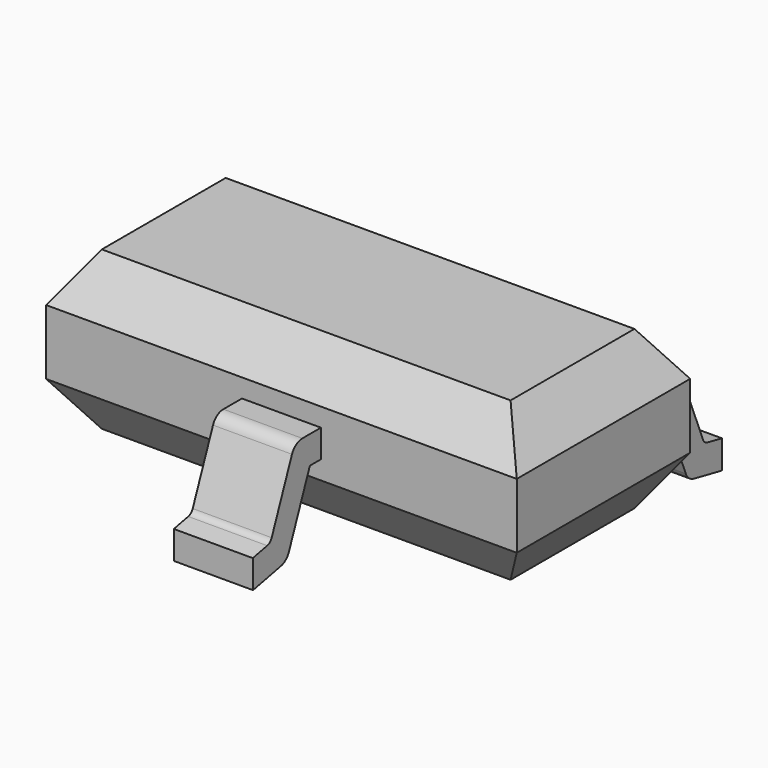
from build123d import *

# Parameters (mm, degrees)
F1_W       = 3.04
F1_H       = 1.4
F2_DEPTH   = 1.02
F3_SIZE2   = 0.3
F3_SIZE    = 0.2
F3_2_SIZE2 = 0.3
F3_2_SIZE  = 0.2
F4_SIZE2   = 0.3
F4_SIZE    = 0.2
F4_2_SIZE2 = 0.3
F4_2_SIZE  = 0.2
F10_DEPTH  = 0.255
F13_DEPTH  = 0.255


# Not quite as in the source:
# - a pattern or mirror of a feature is missing from the dataset's text; its kind, count and spacing are read off the source's solid


with BuildPart() as f2:
    # F1 (on offset) → F2 (new body)
    with BuildSketch(Plane.XY.offset(0.1)):
        Rectangle(F1_W, F1_H)
    extrude(amount=F2_DEPTH)

    # F3
    f3_edges = [f2.edges().sort_by_distance(p)[0] for p in [
        (-1.52, 0, 1.12),
        (1.52, 0, 1.12),
    ]]
    f3_side = f2.faces().sort_by_distance((0, 0, 1.12))[0]
    chamfer(f3_edges, length=F3_SIZE, length2=F3_SIZE2, reference=f3_side)

    # F3#2
    f3_2_edges = [f2.edges().sort_by_distance(p)[0] for p in [
        (-1.52, 0, 0.1),
        (1.52, 0, 0.1),
    ]]
    f3_2_side = f2.faces().sort_by_distance((0, 0, 0.1))[0]
    chamfer(f3_2_edges, length=F3_2_SIZE, length2=F3_2_SIZE2, reference=f3_2_side)

    # F4
    f4_edges = [f2.edges().sort_by_distance(p)[0] for p in [
        (0, -0.7, 1.12),
        (0, 0.7, 1.12),
    ]]
    f4_side = f2.faces().sort_by_distance((0, 0, 1.12))[0]
    chamfer(f4_edges, length=F4_SIZE, length2=F4_SIZE2, reference=f4_side)

    # F4#2
    f4_2_edges = [f2.edges().sort_by_distance(p)[0] for p in [
        (0, -0.7, 0.1),
        (0, 0.7, 0.1),
    ]]
    f4_2_side = f2.faces().sort_by_distance((0, 0, 0.1))[0]
    chamfer(f4_2_edges, length=F4_2_SIZE, length2=F4_2_SIZE2, reference=f4_2_side)

    # F9 (on 3pt) → F10 (join, symmetric)
    with BuildSketch(Plane.YZ):
        with BuildLine():
            Line((-1.25, 0.09), (-1.25, 0))
            ThreePointArc((-1.25, 0), (-1.241013072, 0.0004498178), (-1.2321159768, 0.001794775))
            Line((-1.2321159768, 0.001794775), (-1.0240477755, 0.043981579))
            ThreePointArc((-1.0240477755, 0.043981579), (-0.9843358775, 0.063029665), (-0.9584175942, 0.0986401552))
            Line((-0.9584175942, 0.0986401552), (-0.7913652221, 0.5145161505))
            ThreePointArc((-0.7913652221, 0.5145161505), (-0.7881487587, 0.5185004288), (-0.7832526987, 0.5199999977))
            Line((-0.7832526987, 0.5199999977), (-0.7000000035, 0.5199999977))
            Line((-0.7000000035, 0.5199999977), (-0.7000000035, 0.7))
            Line((-0.7000000035, 0.7), (-0.85, 0.7))
            ThreePointArc((-0.85, 0.7), (-0.9004023889, 0.6845627199), (-0.9335142045, 0.6435466488))
            Line((-0.9335142045, 0.6435466488), (-1.0973164639, 0.2357617917))
            ThreePointArc((-1.0973164639, 0.2357617917), (-1.1117155102, 0.2159781861), (-1.1337776758, 0.2053959161))
            Line((-1.1337776758, 0.2053959161), (-1.25, 0.1818312946))
            Line((-1.25, 0.1818312946), (-1.25, 0.18))
            Line((-1.25, 0.18), (-1.25, 0.09))
        make_face()
    extrude(amount=F10_DEPTH, both=True)

    # F12 (on offset) → F13 (join, symmetric)
    with BuildSketch(Plane.YZ.offset(1.03)):
        with BuildLine():
            Line((1.0240477755, 0.043981579), (1.2321159768, 0.001794775))
            ThreePointArc((1.2321159768, 0.001794775), (1.241013072, 0.0004498178), (1.25, 0))
            Line((1.25, 0), (1.25, 0.1818312946))
            Line((1.25, 0.1818312946), (1.1337776758, 0.2053959161))
            ThreePointArc((1.1337776758, 0.2053959161), (1.1117155102, 0.2159781861), (1.0973164639, 0.2357617917))
            Line((1.0973164639, 0.2357617917), (0.9335142045, 0.6435466488))
            ThreePointArc((0.9335142045, 0.6435466488), (0.9004023889, 0.6845627199), (0.85, 0.7))
            Line((0.85, 0.7), (0.7000000035, 0.7))
            Line((0.7000000035, 0.7), (0.7000000035, 0.5199999977))
            Line((0.7000000035, 0.5199999977), (0.7832526987, 0.5199999977))
            ThreePointArc((0.7832526987, 0.5199999977), (0.7881487587, 0.5185004288), (0.7913652221, 0.5145161505))
            Line((0.7913652221, 0.5145161505), (0.9584175942, 0.0986401552))
            ThreePointArc((0.9584175942, 0.0986401552), (0.9843358775, 0.063029665), (1.0240477755, 0.043981579))
        make_face()
    f13 = extrude(amount=F13_DEPTH, both=True)

    # F13_copies: F13 across plane
    add(f13.mirror(Plane(origin=(0, 0, 0), x_dir=(0, 0, -1), z_dir=(-1, 0, 0))))


solid = f2.part
